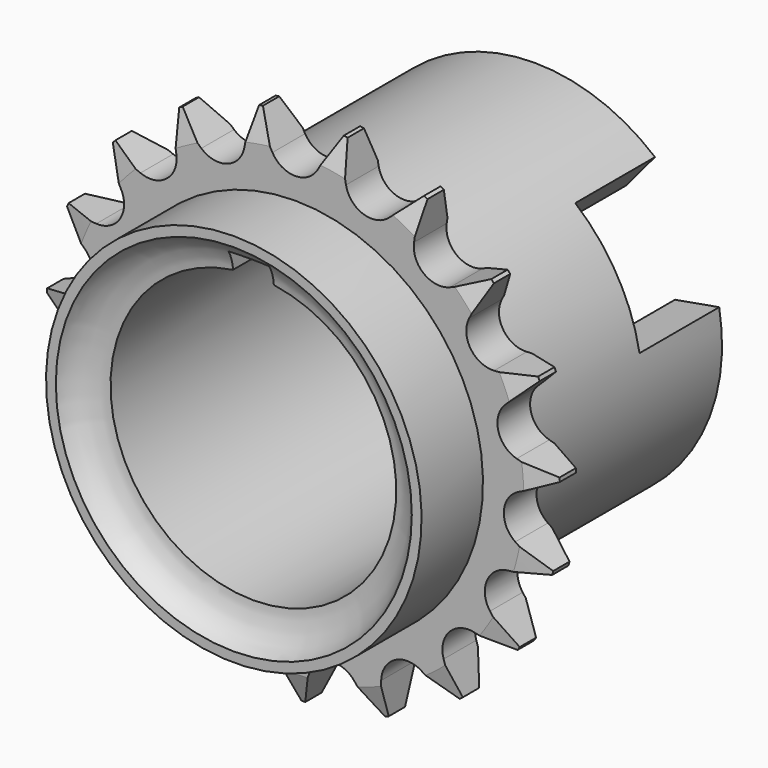
from build123d import *

# Parameters (mm, degrees)
F2_W            = 5
F2_H            = 5
F3_DEPTH        = 46.001
F5_DEPTH        = 12.2
F6_W            = 1.8
F6_H            = 1.8
F7_DEPTH        = 14.4
F9_DEPTH        = 36.6010001
F9_COPIES_COUNT = 19


# Not quite as in the source:
# - a pattern or mirror of a feature is missing from the dataset's text; its kind, count and spacing are read off the source's solid


with BuildPart() as f1:
    # F0 (on Right) → F1 (revolve)
    with BuildSketch(Plane.YZ):
        with BuildLine():
            ThreePointArc((0, 21.8), (2.1088292888, 20.0747646201), (3, 17.5))
            Line((3, 17.5), (46, 17.5))
            Line((46, 17.5), (46, 23))
            Line((46, 23), (14.4, 23))
            Line((14.4, 23), (14.4, 28))
            Line((14.4, 28), (13.15, 31.5))
            Line((13.15, 31.5), (10.65, 31.5))
            Line((10.65, 31.5), (9.4, 28))
            Line((9.4, 28), (9.4, 23))
            Line((9.4, 23), (0, 23))
            Line((0, 23), (0, 21.8))
        make_face()
    revolve(axis=Axis((0, 23, 0), (0, 1, 0)))

    # F2 (on Front) → F3 (cut, through all)
    with BuildSketch(Plane.XZ):
        with Locations((0, 17.1)):
            Rectangle(F2_W, F2_H)
    extrude(amount=-F3_DEPTH, mode=Mode.SUBTRACT)

    # F4 (on face) → F5 (cut)
    with BuildSketch(Plane(origin=(0, 46, 0), x_dir=(-1, 0, 0), z_dir=(0, 1, 0))):
        with BuildLine():
            Line((-22.6505783193, 3.9939080863), (-17.2341356777, 3.0388431092))
            ThreePointArc((-17.2341356777, 3.0388431092), (-15.1554445662, 8.75), (-11.2487831695, 13.4057777546))
            Line((-11.2487831695, 13.4057777546), (-14.7841150228, 17.6190221917))
            ThreePointArc((-14.7841150228, 17.6190221917), (-19.918584287, 11.5), (-22.6505783193, 3.9939080863))
        make_face()
        with BuildLine():
            Line((14.7841150228, 17.6190221917), (11.2487831695, 13.4057777546))
            ThreePointArc((11.2487831695, 13.4057777546), (15.1554445662, 8.75), (17.2341356777, 3.0388431092))
            Line((17.2341356777, 3.0388431092), (22.6505783193, 3.9939080863))
            ThreePointArc((22.6505783193, 3.9939080863), (19.918584287, 11.5), (14.7841150228, 17.6190221917))
        make_face()
        with BuildLine():
            Line((7.8664632965, -21.6129302781), (5.9853525082, -16.4446208638))
            ThreePointArc((5.9853525082, -16.4446208638), (0, -17.5), (-5.9853525082, -16.4446208638))
            Line((-5.9853525082, -16.4446208638), (-7.8664632965, -21.6129302781))
            ThreePointArc((-7.8664632965, -21.6129302781), (0, -23), (7.8664632965, -21.6129302781))
        make_face()
    extrude(amount=-F5_DEPTH, mode=Mode.SUBTRACT)

    # F6 (on face) → F7 (cut)
    with BuildSketch(Plane(origin=(0, 33.8, 0), x_dir=(-1, 0, 0), z_dir=(0, 1, 0))):
        with Locations((0, -22.9)):
            Rectangle(F6_W, F6_H)
    extrude(amount=-F7_DEPTH, mode=Mode.SUBTRACT)

    # F8 (on face) → F9 (cut, through all)
    with BuildSketch(Plane.XZ.offset(-9.4)):
        with BuildLine():
            Line((2.7865500238, 27.2767425624), (4.95, 31.1086402789))
            ThreePointArc((4.95, 31.1086402789), (0, 31.5), (-4.95, 31.1086402789))
            Line((-4.95, 31.1086402789), (-2.7865500238, 27.2767425624))
            ThreePointArc((-2.7865500238, 27.2767425624), (0, 25.65), (2.7865500238, 27.2767425624))
        make_face()
    f9 = extrude(amount=-F9_DEPTH, mode=Mode.SUBTRACT)

    # F9_copies: F9 ×19 about axis
    f9_copies_axis = Axis((0, 0, 0), (0, 1, 0))
    for i in range(1, F9_COPIES_COUNT):
        add(f9.rotate(f9_copies_axis, i * 360 / F9_COPIES_COUNT), mode=Mode.SUBTRACT)


solid = f1.part
